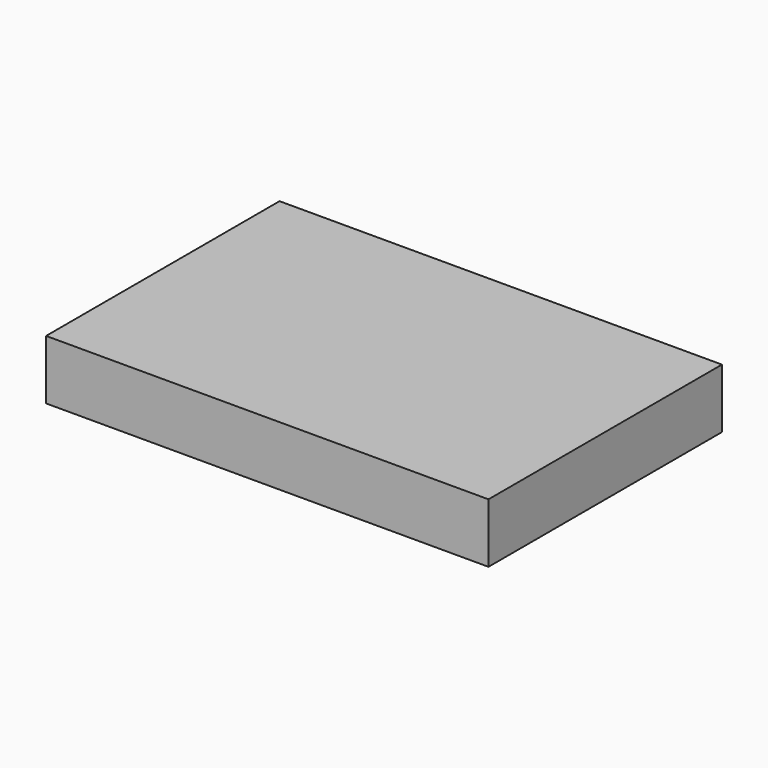
from build123d import *

# Parameters (mm, degrees)
F0_W     = 23.876
F0_H     = 15.748
F1_DEPTH = 3.20802
F3_T     = -1.778
F4_R     = 3.2385
F4_R_2   = 2.6416
F5_DEPTH = 3.06898


# Not quite as in the source:
# - a feature names something its author has since deleted; it is built from what else it names


with BuildPart() as f1:
    # F0 (on Top) → F1 (new body)
    with BuildSketch(Plane.XY):
        with Locations((11.938, 7.874)):
            Rectangle(F0_W, F0_H)
    extrude(amount=F1_DEPTH)

    # F3
    f3_openings = [f1.faces().sort_by_distance(p)[0] for p in [
        (11.938, 7.874, 0),
    ]]
    offset(amount=F3_T, openings=f3_openings)

    # F4 (on face) → F5 (join)
    with BuildSketch(Plane.XY):
        with BuildLine():
            ThreePointArc((4.1275, 7.5388690457), (7.366, 4.3003690457), (10.6045, 7.5388690457))
            ThreePointArc((10.6045, 7.5388690457), (7.366, 10.7773690457), (4.1275, 7.5388690457))
        make_face()
        with BuildLine():
            ThreePointArc((10.0076, 7.5388690457), (7.366, 4.8972690457), (4.7244, 7.5388690457))
            ThreePointArc((4.7244, 7.5388690457), (7.366, 10.1804690457), (10.0076, 7.5388690457))
        make_face(mode=Mode.SUBTRACT)
        with Locations((15.24, 7.5388690457)):
            Circle(F4_R)
        with Locations((15.24, 7.5388690457)):
            Circle(F4_R_2, mode=Mode.SUBTRACT)
    extrude(amount=F5_DEPTH)


solid = f1.part
